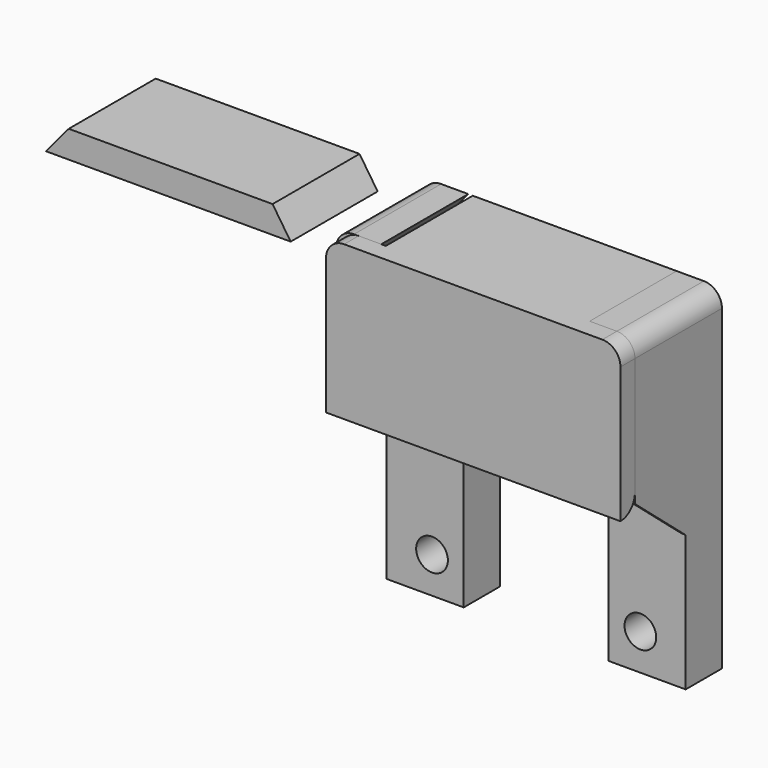
from build123d import *

# Parameters (mm, degrees)
F0_R      = 1.75
F1_DEPTH  = 5
F3_DEPTH  = 5
F5_DEPTH  = 5
F7_DEPTH  = 12.001
F9_DEPTH  = 12
F10_R     = 4.99999
F11_R     = 2
F14_DEPTH = 2
F15_R     = 2
F16_R     = 1.99999


# Not quite as in the source:
# - a fillet or chamfer is up to 0.001 mm smaller than in the source, because OpenCascade refuses the exact size


with BuildPart() as f1:
    # F0 (on Front) → F1 (new body)
    with BuildSketch(Plane.XZ):
        Polygon((-20.7616274655, -1.7146679766), (-15.7616274655, -1.7146679766), (-12.2616274655, -1.7146679766), (-12.2616274655, 13.2853320234), (3.7383725345, 13.2853320234), (3.7383725345, -1.7146679766), (7.2383725345, -1.7146679766), (12.2383725345, -1.7146679766), (12.2383725345, 25.2853320234), (7.2383725345, 25.2853320234), (-15.7616274655, 25.2853320234), (-20.7616274655, 25.2853320234), align=None)
        with Locations((-15.7616274655, 2.2853320234)):
            Circle(F0_R, mode=Mode.SUBTRACT)
        with Locations((7.2383725345, 2.2853320234)):
            Circle(F0_R, mode=Mode.SUBTRACT)
    extrude(amount=F1_DEPTH)

    # F2 (on face) → F3 (join)
    with BuildSketch(Plane(origin=(-20.7616274655, 0, 0), x_dir=(0, -1, 0), z_dir=(-1, 0, 0))):
        Polygon((12, 25.2853320234), (5, 25.2853320234), (5, 13.2853320234), (12, 19.1590294417), align=None)
        Polygon((0, 25.2853320234), (5, 25.2853320234), (12, 25.2853320234), (12, 35.2853320234), (0, 35.2853320234), align=None)
    extrude(amount=-F3_DEPTH)

    # F4 (on face) → F5 (join)
    with BuildSketch(Plane.YZ.offset(12.2383725345)):
        Polygon((-12, 35.2853320234), (-12, 19.1590294417), (-5, 13.2853320234), (-5, 25.2853320234), (0, 25.2853320234), (0, 35.2853320234), align=None)
    extrude(amount=-F5_DEPTH)

    # F6 (on face) → F7 (cut, through all)
    with BuildSketch(Plane(origin=(0, 0, 0), x_dir=(-1, 0, 0), z_dir=(0, 1, 0))):
        Polygon((-7.2383725345, 32.2853320234), (-7.2383725345, 35.2853320234), (-9.2383725345, 32.2853320234), align=None)
        Polygon((15.7616274655, 35.2853320234), (15.7616274655, 32.2853320234), (18.2616274655, 32.2853320234), align=None)
    extrude(amount=-F7_DEPTH, mode=Mode.SUBTRACT)

    # F10 (radius 5 in the source; OpenCascade refuses exactly that, so slightly less here)
    f10_edges = [f1.edges().sort_by_distance(p)[0] for p in [
        (-4.261627, -5, 25.285332),
        (-15.761627, -8.5, 16.222181),
        (7.238373, -8.5, 16.222181),
        (-4.261627, -5, 13.285332),
    ]]
    fillet(f10_edges, radius=F10_R)

    # F11
    f11_edges = [f1.edges().sort_by_distance(p)[0] for p in [
        (-20.761627, -6, 35.285332),
        (12.238373, -6, 35.285332),
    ]]
    fillet(f11_edges, radius=F11_R)


with BuildPart() as f9:
    # F8 (on face) → F9 (new body)
    with BuildSketch(Plane(origin=(0, 0, 0), x_dir=(-1, 0, 0), z_dir=(0, 1, 0))):
        Polygon((15.2616274655, 35.2853320234), (-7.2383725345, 35.2853320234), (-9.2383725345, 32.2853320234), (-7.2383725345, 32.2853320234), (15.7616274655, 32.2853320234), (17.7616274655, 32.2853320234), align=None)
    extrude(amount=-F9_DEPTH)


with BuildPart() as f12_1:
    # F12: copy of F9
    add(f9.part.moved(Location((-35, 0, 0))))


with BuildPart() as f9_1:
    add(f9.part)

    # F13 (on face) → F14 (join)
    with BuildSketch(Plane.XZ.offset(12)):
        Polygon((12.2383725345, 35.2853320234), (7.2383725345, 35.2853320234), (9.2383725345, 32.2853320234), (-17.7616274655, 32.2853320234), (-15.2616274655, 35.2853320234), (-20.2616274655, 35.2853320234), (-20.2616274655, 18.2853320234), (12.2383725345, 18.2853320234), align=None)
        Polygon((7.2383725345, 35.2853320234), (-4.0116274655, 35.2853320234), (-15.2616274655, 35.2853320234), (-17.7616274655, 32.2853320234), (9.2383725345, 32.2853320234), align=None)
    extrude(amount=F14_DEPTH)

    # F15
    f15_edges = [f9_1.edges().sort_by_distance(p)[0] for p in [
        (12.238373, -13, 35.285332),
        (-20.261627, -13, 35.285332),
    ]]
    fillet(f15_edges, radius=F15_R)

    # F16 (radius 2 in the source; OpenCascade refuses exactly that, so slightly less here)
    f16_edges = [f9_1.edges().sort_by_distance(p)[0] for p in [
        (-4.011627, -12, 18.285332),
    ]]
    fillet(f16_edges, radius=F16_R)


solid = Compound([f1.part, f12_1.part, f9_1.part])
